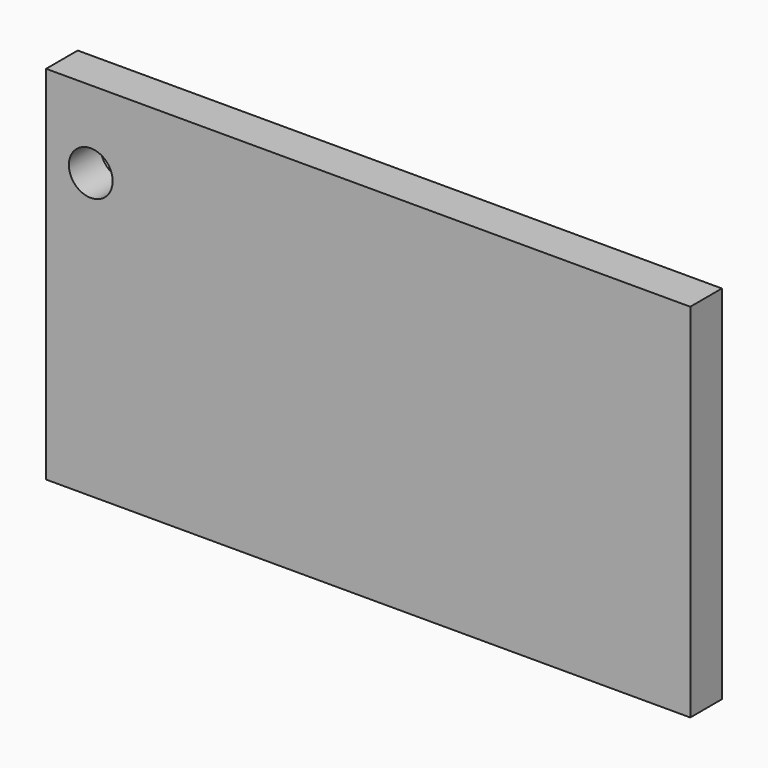
from build123d import *

# Parameters (mm, degrees)
F1_W     = 5.1343291998
F1_H     = 4.8490911722
F2_DEPTH = 12.7
F0_R     = 7.0231
F3_DEPTH = 25.4


with BuildPart() as f2:
    # F1 (on Front) → F2 (new body)
    with BuildSketch(Plane.XZ):
        Polygon((103.5248413682, 57.333368808), (-103.27462852, 57.333368808), (-103.27462852, -58.7595701218), (103.5248413682, -58.7595701218), (103.5248413682, -58.4743283689), (98.3905121684, -58.4743283689), (98.3905121684, -53.6252371967), (103.5248413682, -53.6252371967), align=None)
        with Locations((100.9576767683, -56.0497827828)):
            Rectangle(F1_W, F1_H)
    extrude(amount=F2_DEPTH)

    # F0 (on Front) → F3 (cut)
    with BuildSketch(Plane.XZ):
        with Locations((-88.9342725277, 32.5196869671)):
            Circle(F0_R)
    extrude(amount=F3_DEPTH, mode=Mode.SUBTRACT)


solid = f2.part
